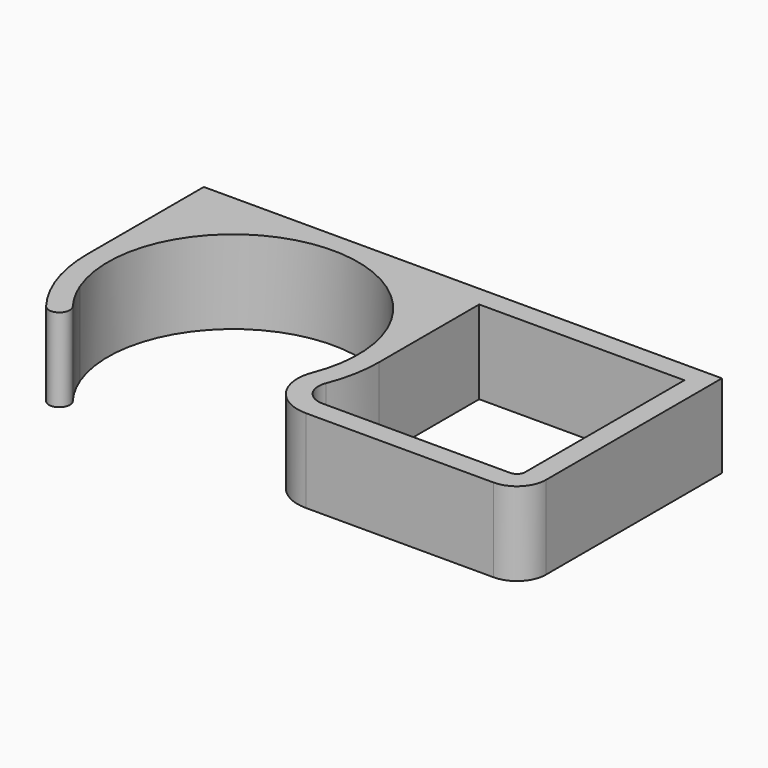
from build123d import *

# Parameters (mm, degrees)
F1_DEPTH = 12.7
F2_DEPTH = 12.7
F3_DEPTH = 12.7
F4_W     = 6.35
F4_H     = 25.4
F5_DEPTH = 62.464519896


# Not quite as in the source:
# - a feature names something its author has since deleted; it is built from what else it names


with BuildPart() as f1:
    # F0 (on Top) → F1 (new body, symmetric)
    with BuildSketch(Plane.XY):
        with BuildLine():
            ThreePointArc((-35.5333842184, -13.7473126824), (0.1257546156, 38.0997924637), (35.4418604651, -13.9815781216))
            ThreePointArc((35.4418604651, -13.9815781216), (36.7563215678, -25.7870785948), (47.2558139535, -31.3421041622))
            Line((47.2558139535, -31.3421041622), (104.4058139535, -31.3421041622))
            ThreePointArc((104.4058139535, -31.3421041622), (110.669864998, -28.7474492641), (113.264519896, -22.4833982196))
            Line((113.264519896, -22.4833982196), (113.264519896, 44.45))
            Line((113.264519896, 44.45), (106.914519896, 44.45))
            Line((106.914519896, 44.45), (106.914519896, -22.4833982196))
            ThreePointArc((106.914519896, -22.4833982196), (106.1797369375, -24.2573212036), (104.4058139535, -24.9921041622))
            Line((104.4058139535, -24.9921041622), (47.2558139535, -24.9921041622))
            ThreePointArc((47.2558139535, -24.9921041622), (42.0060677606, -22.2145913785), (41.3488372093, -16.3118411419))
            ThreePointArc((41.3488372093, -16.3118411419), (43.6678274818, -8.3020083729), (44.45, 0))
            ThreePointArc((44.45, 0), (31.4308965011, 31.4308963464), (2.188e-07, 44.45))
            ThreePointArc((2.188e-07, 44.45), (-31.4308963464, 31.4308965011), (-44.45, 0))
            ThreePointArc((-44.45, 0), (-43.6949916081, -8.157831107), (-41.4556149214, -16.0385314629))
            ThreePointArc((-41.4556149214, -16.0385314629), (-41.4024515906, -16.1752744115), (-41.3488372093, -16.3118411419))
            ThreePointArc((-41.3488372093, -16.3118411419), (-38.7334132864, -21.806540193), (-35.3920150029, -26.8925226418))
            ThreePointArc((-35.3920150029, -26.8925226418), (-30.9431194568, -27.499629239), (-30.3360128596, -23.0507336929))
            ThreePointArc((-30.3360128596, -23.0507336929), (-33.2615811181, -18.581636675), (-35.5333842184, -13.7473126825))
        make_face()
    extrude(amount=F1_DEPTH, both=True)

    # F0 (on Top) → F2 (join, symmetric)
    with BuildSketch(Plane.XY):
        with BuildLine():
            Line((44.45, 0), (44.45, 44.45))
            Line((44.45, 44.45), (2.188e-07, 44.45))
            ThreePointArc((2.188e-07, 44.45), (31.4308965011, 31.4308963464), (44.45, 0))
        make_face()
    extrude(amount=F2_DEPTH, both=True)

    # F0 (on Top) → F3 (join, symmetric)
    with BuildSketch(Plane.XY):
        with BuildLine():
            Line((-44.45, 44.45), (-44.45, 0))
            ThreePointArc((-44.45, 0), (-31.4308963464, 31.4308965011), (2.188e-07, 44.45))
            Line((2.188e-07, 44.45), (-44.45, 44.45))
        make_face()
    extrude(amount=F3_DEPTH, both=True)

    # F4 (on face) → F5 (join, through all)
    with BuildSketch(Plane(origin=(106.914519896, 0, 0), x_dir=(0, -1, 0), z_dir=(-1, 0, 0))):
        with Locations((-41.275, 0)):
            Rectangle(F4_W, F4_H)
    extrude(amount=F5_DEPTH)


solid = f1.part
